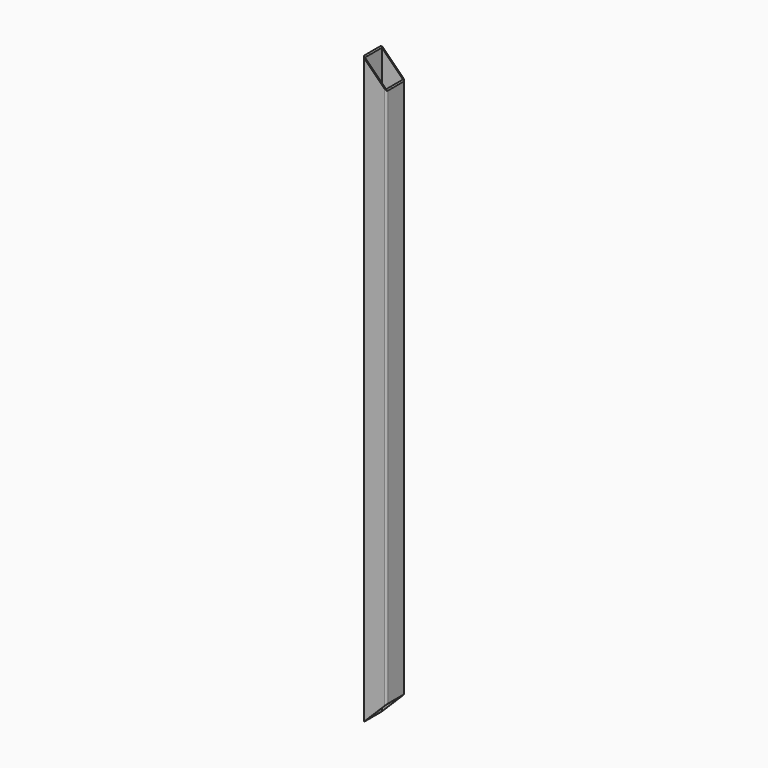
from build123d import *

# Parameters (mm, degrees)
F0_W     = 36
F0_H     = 36
F1_DEPTH = 500
F3_DEPTH = 40.001


# Not quite as in the source:
# - a pattern or mirror of a feature is missing from the dataset's text; its kind, count and spacing are read off the source's solid


with BuildPart() as f1:
    # F0 (on Top) → F1 (new body, symmetric)
    with BuildSketch(Plane.XY):
        with BuildLine():
            Line((17, 20), (-17, 20))
            ThreePointArc((-17, 20), (-19.1213203436, 19.1213203436), (-20, 17))
            Line((-20, 17), (-20, -17))
            ThreePointArc((-20, -17), (-19.1213203436, -19.1213203436), (-17, -20))
            Line((-17, -20), (17, -20))
            ThreePointArc((17, -20), (19.1213203436, -19.1213203436), (20, -17))
            Line((20, -17), (20, 17))
            ThreePointArc((20, 17), (19.1213203436, 19.1213203436), (17, 20))
        make_face()
        Rectangle(F0_W, F0_H, mode=Mode.SUBTRACT)
    extrude(amount=F1_DEPTH, both=True)

    # F2 (on face) → F3 (cut, through all)
    with BuildSketch(Plane.XZ.offset(20)):
        Polygon((20, 500), (-20, 500), (20, 460), align=None)
    f3 = extrude(amount=-F3_DEPTH, mode=Mode.SUBTRACT)

    # F3_copies: F3 across plane
    add(f3.mirror(Plane(origin=(0, 0, 0), x_dir=(-1, 0, 0), z_dir=(0, 0, -1))), mode=Mode.SUBTRACT)


solid = f1.part
